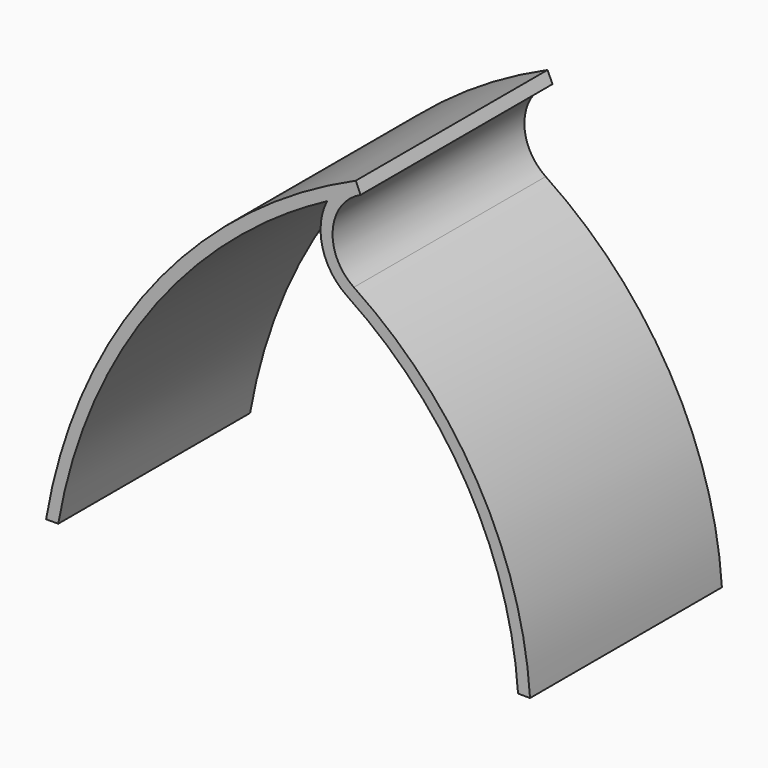
from build123d import *

# Parameters (mm, degrees)
F1_DEPTH      = 200
F1_DEPTH_BACK = 200
F2_T1_DEPTH   = 400
F4_DEPTH      = 400


# Not quite as in the source:
# - a fillet or chamfer that OpenCascade refuses, or shapes differently, is made with other operations: its cross-section is extruded or revolved along the edge and cut away or added


with BuildPart() as f1:
    # F0 (on Front) → F1 (new body, two sides)
    with BuildSketch(Plane.XZ) as f1_sk:
        with BuildLine():
            Line((524.5966985083, 646.8509630198), (516.4602606489, 665.1211129634))
            ThreePointArc((516.4602606489, 665.1211129634), (174.8026570637, 397.3412013082), (0, 0))
            Line((0, 0), (20.2946136834, 0))
            ThreePointArc((20.2946136834, 0), (140.429327731, 313.2929945553), (369.9696430546, 558.0297788724))
            ThreePointArc((369.9696430546, 558.0297788724), (661.1169981621, 340.7216012774), (787.2059225715, 0))
            Line((787.2059225715, 0), (807.2493330572, 0))
            ThreePointArc((807.2493330572, 0), (681.631739827, 346.6110161721), (389.7878488942, 571.8800100128))
            ThreePointArc((389.7878488942, 571.8800100128), (455.5312679724, 612.3522202116), (524.5966985083, 646.8509630198))
        make_face()
    extrude(amount=F1_DEPTH)
    extrude(f1_sk.sketch, amount=-F1_DEPTH_BACK)

    # F2: fillet of radius 80 on 1 edges, made by hand

    # F2_s2 → F2_t1 (join)
    with BuildSketch(Plane.XZ.offset(-200)):
        with BuildLine():
            ThreePointArc((524.5965325964, 646.8513269885), (478.0294026942, 580.3882007889), (513.5263540919, 507.4100453379))
            Line((513.5263540919, 507.4100453379), (509.1010667383, 500.7453599443))
            ThreePointArc((509.1010667383, 500.7453599443), (449.6679775139, 535.8272349913), (386.8614602924, 564.434377111))
            Line((386.8614602924, 564.434377111), (385.2964579687, 578.5003277629))
            ThreePointArc((385.2964579687, 578.5003277629), (451.6430451413, 619.3438525513), (521.2782630933, 654.13076976))
            Line((521.2782630933, 654.13076976), (524.5965325964, 646.8513269885))
        make_face()
    extrude(amount=F2_T1_DEPTH)

    # F3 (on face) → F4 (cut, through all)
    with BuildSketch(Plane(origin=(0, 200, 0), x_dir=(-1, 0, 0), z_dir=(0, 1, 0))):
        with BuildLine():
            ThreePointArc((-468.7201479158, 619.5389112196), (-461.0435334952, 548.7124418966), (-502.4630068664, 490.7491225353))
            ThreePointArc((-502.4630068664, 490.7491225353), (-438.1743029198, 528.2452259031), (-369.9696430546, 558.0297788724))
            ThreePointArc((-369.9696430546, 558.0297788724), (-418.3179553497, 590.4330572448), (-468.7201479158, 619.5389112196))
        make_face()
    extrude(amount=-F4_DEPTH, mode=Mode.SUBTRACT)


solid = f1.part
